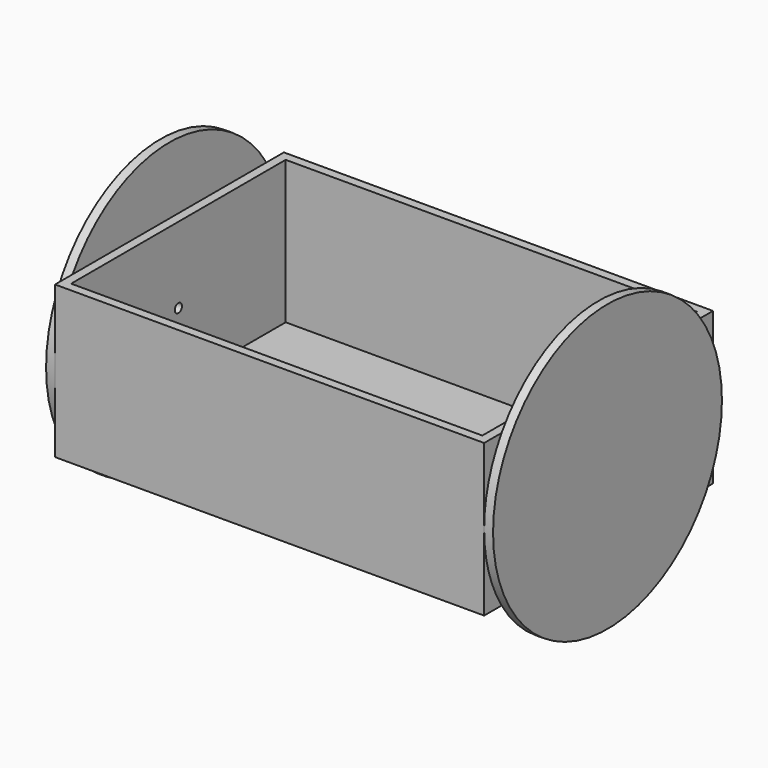
from build123d import *

# Parameters (mm, degrees)
F0_W      = 152.4
F0_H      = 101.6
F1_DEPTH  = 3.175
F2_W      = 146.05
F2_H      = 3.175
F3_DEPTH  = 50.8
F5_DEPTH  = 25.4
F7_DEPTH  = 3.175
F8_DEPTH  = 25.4
F9_R      = 50.8
F10_DEPTH = 3.175
F11_R     = 50.8
F12_DEPTH = 3.175


# Not quite as in the source:
# - a length typed as a fraction of an inch, garbled in the dataset ("3 / 203.2 mm" for 3/8 in), is restored


with BuildPart() as f1:
    # F0 (on Top) → F1 (new body)
    with BuildSketch(Plane.XY):
        Rectangle(F0_W, F0_H)
    extrude(amount=F1_DEPTH)

    # F2 (on face) → F3 (join)
    with BuildSketch(Plane.XY.offset(3.175)):
        Polygon((-73.025, 50.8), (-76.2, 50.8), (-76.2, -50.8), (-73.025, -50.8), (-73.025, -47.625), (-73.025, 47.625), align=None)
        with Locations((0, 49.2125)):
            Rectangle(F2_W, F2_H)
        Polygon((76.2, 50.8), (73.025, 50.8), (73.025, 47.625), (73.025, -47.625), (73.025, -50.8), (76.2, -50.8), align=None)
        with Locations((0, -49.2125)):
            Rectangle(F2_W, F2_H)
    extrude(amount=F3_DEPTH)

    # F4 (on face) → F5 (cut)
    with BuildSketch(Plane.YZ.offset(76.2)):
        with BuildLine():
            ThreePointArc((1.5875, 26.9875), (0, 28.575), (-1.5875, 26.9875))
            Line((-1.5875, 26.9875), (1.5875, 26.9875))
        make_face()
        with BuildLine():
            Line((1.5875, 26.9875), (-1.5875, 26.9875))
            ThreePointArc((-1.5875, 26.9875), (0, 25.4), (1.5875, 26.9875))
        make_face()
    extrude(amount=-F5_DEPTH, mode=Mode.SUBTRACT)

    # F6 (on face) → F7 (cut)
    with BuildSketch(Plane(origin=(-76.2, 0, 0), x_dir=(0, -1, 0), z_dir=(-1, 0, 0))):
        with BuildLine():
            Line((-1.5875, 26.9875), (1.5875, 26.9875))
            ThreePointArc((1.5875, 26.9875), (0, 28.575), (-1.5875, 26.9875))
        make_face()
        with BuildLine():
            ThreePointArc((-1.5875, 26.9875), (0, 25.4), (1.5875, 26.9875))
            Line((1.5875, 26.9875), (-1.5875, 26.9875))
        make_face()
    extrude(amount=F7_DEPTH, mode=Mode.SUBTRACT)

    # F6 (on face) → F8 (cut)
    with BuildSketch(Plane(origin=(-76.2, 0, 0), x_dir=(0, -1, 0), z_dir=(-1, 0, 0))):
        with BuildLine():
            Line((-1.5875, 26.9875), (1.5875, 26.9875))
            ThreePointArc((1.5875, 26.9875), (0, 28.575), (-1.5875, 26.9875))
        make_face()
        with BuildLine():
            ThreePointArc((-1.5875, 26.9875), (0, 25.4), (1.5875, 26.9875))
            Line((1.5875, 26.9875), (-1.5875, 26.9875))
        make_face()
    extrude(amount=-F8_DEPTH, mode=Mode.SUBTRACT)

    # F9 (on face) → F10 (join)
    with BuildSketch(Plane.YZ.offset(76.2)):
        with Locations((0, 26.9875)):
            Circle(F9_R)
    extrude(amount=F10_DEPTH)

    # F11 (on face) → F12 (join)
    with BuildSketch(Plane(origin=(-76.2, 0, 0), x_dir=(0, -1, 0), z_dir=(-1, 0, 0))):
        with Locations((0, 26.9875)):
            Circle(F11_R)
    extrude(amount=F12_DEPTH)


solid = f1.part
